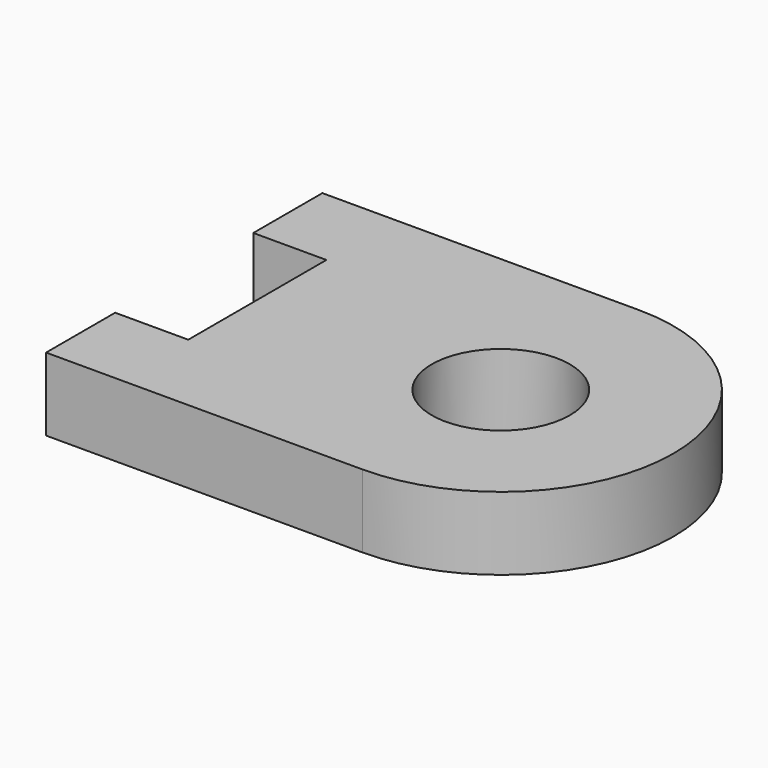
from build123d import *

# Parameters (mm, degrees)
F0_R     = 6
F1_DEPTH = 6.35


# Not quite as in the source:
# - a feature names something its author has since deleted; it is built from what else it names


with BuildPart() as f1:
    # F0 (on Top) → F1 (new body)
    with BuildSketch(Plane.XY):
        with BuildLine():
            Line((-27.5, 15), (-27.5, 7.5))
            Line((-27.5, 7.5), (-21.15, 7.5))
            Line((-21.15, 7.5), (-21.15, -7.5))
            Line((-21.15, -7.5), (-27.5, -7.5))
            Line((-27.5, -7.5), (-27.5, -15))
            Line((-27.5, -15), (3.27e-08, -15))
            ThreePointArc((3.27e-08, -15), (-15, -1.63e-08), (0, 15))
            Line((0, 15), (-27.5, 15))
        make_face()
        with BuildLine():
            ThreePointArc((15, 0), (10.6066017178, 10.6066017178), (0, 15))
            ThreePointArc((0, 15), (-15, -1.63e-08), (3.27e-08, -15))
            ThreePointArc((3.27e-08, -15), (10.6066017294, -10.6066017062), (15, 0))
        make_face()
        Circle(F0_R, mode=Mode.SUBTRACT)
    extrude(amount=F1_DEPTH)


solid = f1.part
